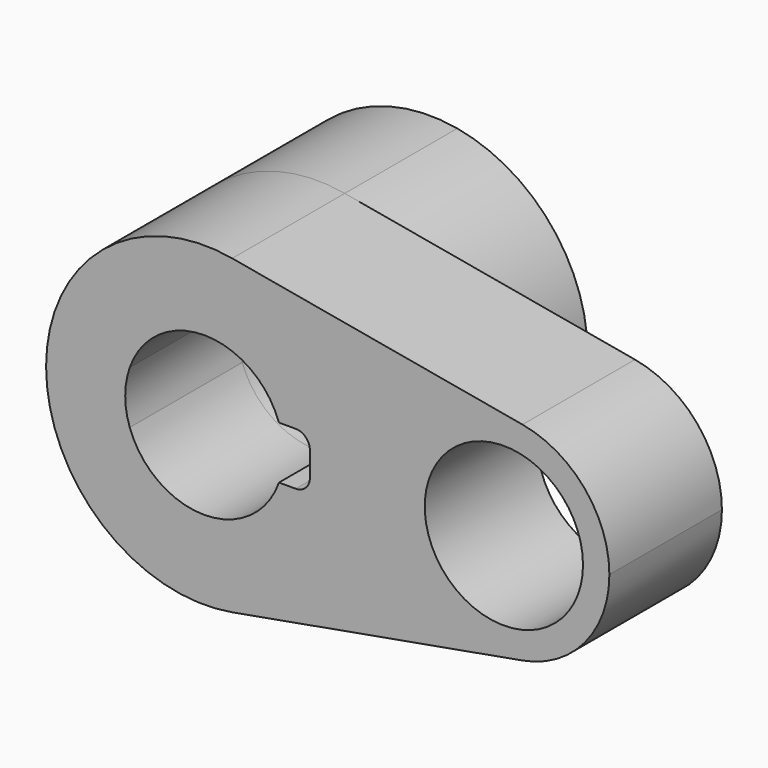
from build123d import *
from build123d import SkipClean  # not in build123d's __all__

# Parameters (mm, degrees)
F0_R     = 0.5625
F1_DEPTH = 1
F2_R     = 0.1
F3_DEPTH = 1
F4_R     = 0.1


with BuildPart() as f1:
    # F0 (on Front) → F1 (new body)
    with BuildSketch(Plane.XZ):
        with BuildLine():
            ThreePointArc((-11.8420327247, 1.107410961), (-11.1774751155, 0.7220453715), (-10.9151891362, 0))
            ThreePointArc((-10.9151891362, 0), (-11.1774751155, -0.7220453715), (-11.8420327247, -1.107410961))
            Line((-11.8420327247, -1.107410961), (-9.7790848619, -0.738273974))
            ThreePointArc((-9.7790848619, -0.738273974), (-10.6611891362, 0), (-9.7790848619, 0.738273974))
            Line((-9.7790848619, 0.738273974), (-11.8420327247, 1.107410961))
        make_face()
        with BuildLine():
            ThreePointArc((-9.1611891362, 0), (-9.3360464557, 0.481363581), (-9.7790848619, 0.738273974))
            ThreePointArc((-9.7790848619, 0.738273974), (-10.6611891362, 0), (-9.7790848619, -0.738273974))
            ThreePointArc((-9.7790848619, -0.738273974), (-9.3360464557, -0.481363581), (-9.1611891362, 0))
        make_face()
        with Locations((-9.9111891362, 0)):
            Circle(F0_R, mode=Mode.SUBTRACT)
        with BuildLine():
            ThreePointArc((-11.8420327247, -1.107410961), (-11.1774751155, -0.7220453715), (-10.9151891362, 0))
            ThreePointArc((-10.9151891362, 0), (-11.1774751155, 0.7220453715), (-11.8420327247, 1.107410961))
            ThreePointArc((-11.8420327247, 1.107410961), (-13.1651891362, 0), (-11.8420327247, -1.107410961))
        make_face()
        with BuildLine():
            ThreePointArc((-12.5705192221, 0.1875), (-12.0401891362, 0.5625), (-11.5098590503, 0.1875))
            Line((-11.5098590503, 0.1875), (-11.2901891362, 0.1875))
            Line((-11.2901891362, 0.1875), (-11.2901891362, -0.1875))
            Line((-11.2901891362, -0.1875), (-11.5098590503, -0.1875))
            ThreePointArc((-11.5098590503, -0.1875), (-12.0401891362, -0.5625), (-12.5705192221, -0.1875))
            Line((-12.5705192221, -0.1875), (-12.7901891362, -0.1875))
            Line((-12.7901891362, -0.1875), (-12.7901891362, 0.1875))
            Line((-12.7901891362, 0.1875), (-12.5705192221, 0.1875))
        make_face(mode=Mode.SUBTRACT)
        with BuildLine():
            ThreePointArc((-12.5705192221, -0.1875), (-12.6026891362, 0), (-12.5705192221, 0.1875))
            Line((-12.5705192221, 0.1875), (-12.7901891362, 0.1875))
            Line((-12.7901891362, 0.1875), (-12.7901891362, -0.1875))
            Line((-12.7901891362, -0.1875), (-12.5705192221, -0.1875))
        make_face()
    extrude(amount=F1_DEPTH)

    # F2
    f2_edges = [f1.edges().sort_by_distance(p)[0] for p in [
        (-11.290189, -0.5, 0.1875),
        (-11.290189, -0.5, -0.1875),
    ]]
    fillet(f2_edges, radius=F2_R)

    # F0 (on Front) → F3 (join)
    with BuildSketch(Plane.XZ):
        with BuildLine():
            ThreePointArc((-11.8420327247, -1.107410961), (-11.1774751155, -0.7220453715), (-10.9151891362, 0))
            ThreePointArc((-10.9151891362, 0), (-11.1774751155, 0.7220453715), (-11.8420327247, 1.107410961))
            ThreePointArc((-11.8420327247, 1.107410961), (-13.1651891362, 0), (-11.8420327247, -1.107410961))
        make_face()
        with BuildLine():
            ThreePointArc((-12.5705192221, 0.1875), (-12.0401891362, 0.5625), (-11.5098590503, 0.1875))
            Line((-11.5098590503, 0.1875), (-11.2901891362, 0.1875))
            Line((-11.2901891362, 0.1875), (-11.2901891362, -0.1875))
            Line((-11.2901891362, -0.1875), (-11.5098590503, -0.1875))
            ThreePointArc((-11.5098590503, -0.1875), (-12.0401891362, -0.5625), (-12.5705192221, -0.1875))
            Line((-12.5705192221, -0.1875), (-12.7901891362, -0.1875))
            Line((-12.7901891362, -0.1875), (-12.7901891362, 0.1875))
            Line((-12.7901891362, 0.1875), (-12.5705192221, 0.1875))
        make_face(mode=Mode.SUBTRACT)
        with BuildLine():
            ThreePointArc((-12.5705192221, -0.1875), (-12.6026891362, 0), (-12.5705192221, 0.1875))
            Line((-12.5705192221, 0.1875), (-12.7901891362, 0.1875))
            Line((-12.7901891362, 0.1875), (-12.7901891362, -0.1875))
            Line((-12.7901891362, -0.1875), (-12.5705192221, -0.1875))
        make_face()
    with SkipClean():  # cleaning this boolean's faces spoils the solid; the shape is the same uncleaned
        extrude(amount=-F3_DEPTH)

    # F4
    f4_edges = [f1.edges().sort_by_distance(p)[0] for p in [
        (-11.290189, 0.5, 0.1875),
        (-11.290189, 0.5, -0.1875),
    ]]
    fillet(f4_edges, radius=F4_R)


solid = f1.part
